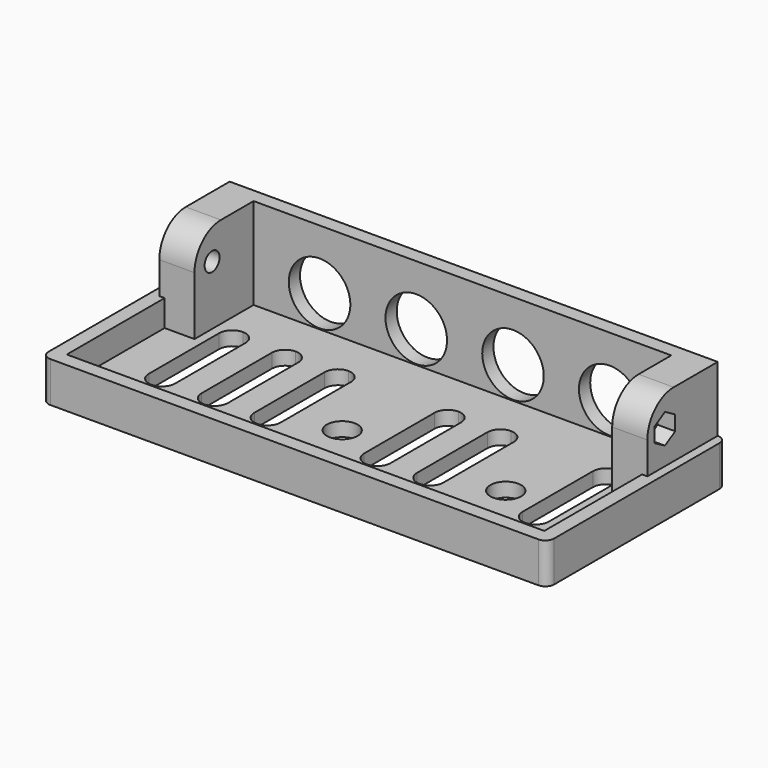
from build123d import *

# Parameters (mm, degrees)
F0_W      = 115
F0_H      = 51
F0_R      = 3.5
F1_DEPTH  = 3.2
F3_DEPTH  = 24
F5_DEPTH  = 6
F6_R      = 2.125
F7_DEPTH  = 113.001
F8_R      = 7.5
F9_R      = 2
F10_R     = 7
F11_DEPTH = 5
F13_DEPTH = 4


# Not quite as in the source:
# - a pattern or mirror of a feature is missing from the dataset's text; its kind, count and spacing are read off the source's solid


with BuildPart() as f1:
    # F0 (on Top) → F1 (new body)
    with BuildSketch(Plane.XY):
        Rectangle(F0_W, F0_H)
        with BuildLine():
            Line((-39.5, 10), (-39.5, -10))
            ThreePointArc((-39.5, -10), (-40.3786796564, -12.1213203436), (-42.5, -13))
            ThreePointArc((-42.5, -13), (-44.6213203436, -12.1213203436), (-45.5, -10))
            Line((-45.5, -10), (-45.5, 10))
            ThreePointArc((-45.5, 10), (-44.6213203436, 12.1213203436), (-42.5, 13))
            ThreePointArc((-42.5, 13), (-40.3786796564, 12.1213203436), (-39.5, 10))
        make_face(mode=Mode.SUBTRACT)
        with Locations((-5.112, -5.5)):
            Circle(F0_R, mode=Mode.SUBTRACT)
        with Locations((32.1, -5.5)):
            Circle(F0_R, mode=Mode.SUBTRACT)
        with BuildLine():
            Line((-27.5, 10), (-27.5, -10))
            ThreePointArc((-27.5, -10), (-28.3786796564, -12.1213203436), (-30.5, -13))
            ThreePointArc((-30.5, -13), (-32.6213203436, -12.1213203436), (-33.5, -10))
            Line((-33.5, -10), (-33.5, 10))
            ThreePointArc((-33.5, 10), (-32.6213203436, 12.1213203436), (-30.5, 13))
            ThreePointArc((-30.5, 13), (-28.3786796564, 12.1213203436), (-27.5, 10))
        make_face(mode=Mode.SUBTRACT)
        with BuildLine():
            Line((-15.5, 10), (-15.5, -10))
            ThreePointArc((-15.5, -10), (-16.3786796564, -12.1213203436), (-18.5, -13))
            ThreePointArc((-18.5, -13), (-20.6213203436, -12.1213203436), (-21.5, -10))
            Line((-21.5, -10), (-21.5, 10))
            ThreePointArc((-21.5, 10), (-20.6213203436, 12.1213203436), (-18.5, 13))
            ThreePointArc((-18.5, 13), (-16.3786796564, 12.1213203436), (-15.5, 10))
        make_face(mode=Mode.SUBTRACT)
        with BuildLine():
            Line((9.5, 10), (9.5, -10))
            ThreePointArc((9.5, -10), (8.6213203436, -12.1213203436), (6.5, -13))
            ThreePointArc((6.5, -13), (4.3786796564, -12.1213203436), (3.5, -10))
            Line((3.5, -10), (3.5, 10))
            ThreePointArc((3.5, 10), (4.3786796564, 12.1213203436), (6.5, 13))
            ThreePointArc((6.5, 13), (8.6213203436, 12.1213203436), (9.5, 10))
        make_face(mode=Mode.SUBTRACT)
        with BuildLine():
            Line((21.5, 10), (21.5, -10))
            ThreePointArc((21.5, -10), (20.6213203436, -12.1213203436), (18.5, -13))
            ThreePointArc((18.5, -13), (16.3786796564, -12.1213203436), (15.5, -10))
            Line((15.5, -10), (15.5, 10))
            ThreePointArc((15.5, 10), (16.3786796564, 12.1213203436), (18.5, 13))
            ThreePointArc((18.5, 13), (20.6213203436, 12.1213203436), (21.5, 10))
        make_face(mode=Mode.SUBTRACT)
        with BuildLine():
            Line((45.5, 10), (45.5, -10))
            ThreePointArc((45.5, -10), (44.6213203436, -12.1213203436), (42.5, -13))
            ThreePointArc((42.5, -13), (40.3786796564, -12.1213203436), (39.5, -10))
            Line((39.5, -10), (39.5, 10))
            ThreePointArc((39.5, 10), (40.3786796564, 12.1213203436), (42.5, 13))
            ThreePointArc((42.5, 13), (44.6213203436, 12.1213203436), (45.5, 10))
        make_face(mode=Mode.SUBTRACT)
    extrude(amount=F1_DEPTH)

    # F2 (on face) → F3 (join)
    with BuildSketch(Plane(origin=(0, 0, 0), x_dir=(1, 0, 0), z_dir=(0, 0, -1))):
        Polygon((-47.5, -5.5), (-55.5, -5.5), (-55.5, -25.5), (55.5, -25.5), (55.5, -5.5), (47.5, -5.5), (47.5, -22.3), (-47.5, -22.3), align=None)
    extrude(amount=-F3_DEPTH)

    # F4 (on face) → F5 (join)
    with BuildSketch(Plane.XY.offset(3.2)):
        Polygon((-55.5, 5.5), (-55.5, 25.5), (-57.5, 25.5), (-57.5, -25.5), (57.5, -25.5), (57.5, 25.5), (55.5, 25.5), (55.5, 5.5), (54.3, 5.5), (54.3, -22.3), (-54.3, -22.3), (-54.3, 5.5), align=None)
    extrude(amount=F5_DEPTH)

    # F6 (on face) → F7 (cut, through all)
    with BuildSketch(Plane.YZ.offset(55.5)):
        with Locations((10.5, 16.7)):
            Circle(F6_R)
    extrude(amount=-F7_DEPTH, mode=Mode.SUBTRACT)

    # F8
    f8_edges = [f1.edges().sort_by_distance(p)[0] for p in [
        (51.5, 5.5, 24),
        (-51.5, 5.5, 24),
    ]]
    fillet(f8_edges, radius=F8_R)

    # F9
    f9_edges = [f1.edges().sort_by_distance(p)[0] for p in [
        (-57.5, -25.5, 4.6),
        (57.5, -25.5, 4.6),
        (57.5, 25.5, 4.6),
        (-57.5, 25.5, 4.6),
    ]]
    fillet(f9_edges, radius=F9_R)

    # F10 (on face) → F11 (cut)
    with BuildSketch(Plane(origin=(0, 25.5, 0), x_dir=(-1, 0, 0), z_dir=(0, 1, 0))):
        with Locations((-33.5, 10.4)):
            Circle(F10_R)
        with Locations((-11.5, 10.4)):
            Circle(F10_R)
        with Locations((10.5, 10.4)):
            Circle(F10_R)
        with Locations((32.5, 10.4)):
            Circle(F10_R)
    extrude(amount=-F11_DEPTH, mode=Mode.SUBTRACT)

    # F12 (on face) → F13 (cut)
    with BuildSketch(Plane(origin=(-55.5, 0, 0), x_dir=(0, -1, 0), z_dir=(-1, 0, 0))):
        Polygon((-7.575, 15.0112504626), (-7.575, 18.3887495374), (-10.5, 20.0774990748), (-13.425, 18.3887495374), (-13.425, 15.0112504626), (-10.5, 13.3225009252), align=None)
    f13 = extrude(amount=-F13_DEPTH, mode=Mode.SUBTRACT)

    # F13_copies: F13 across plane
    add(f13.mirror(Plane(origin=(0, 0, 0), x_dir=(0, 0, 1), z_dir=(1, 0, 0))), mode=Mode.SUBTRACT)


solid = f1.part
